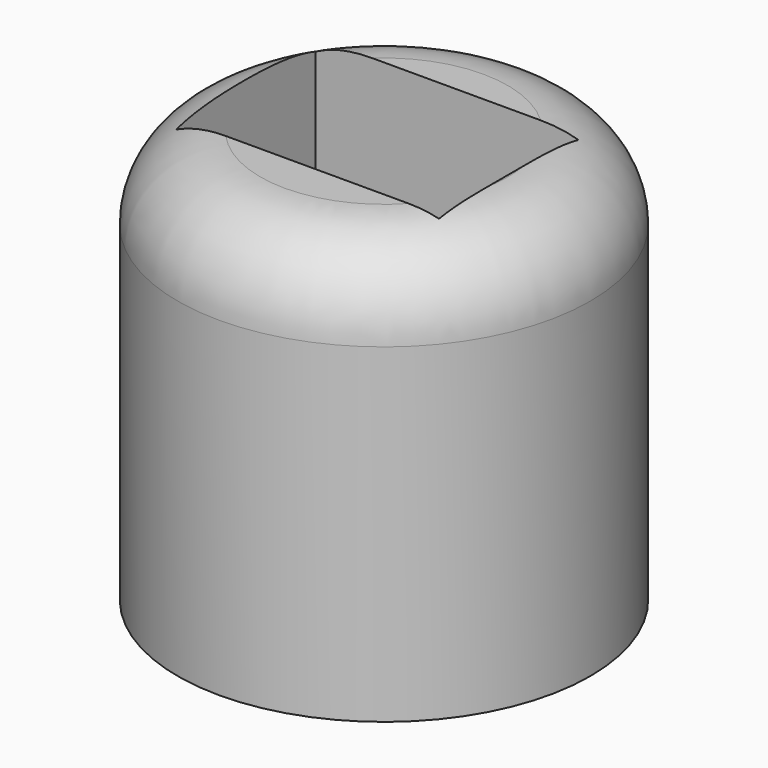
from build123d import *

# Parameters (mm, degrees)
F0_R     = 12.5
F1_DEPTH = 25
F2_W     = 15.9198134206
F2_H     = 10.5606685393
F3_DEPTH = 25


# Not quite as in the source:
# - a fillet or chamfer that OpenCascade refuses, or shapes differently, is made with other operations: its cross-section is extruded or revolved along the edge and cut away or added


with BuildPart() as f1:
    # F0 (on Top) → F1 (new body)
    with BuildSketch(Plane.XY):
        Circle(F0_R)
    extrude(amount=F1_DEPTH)

    # F2 (on face) → F3 (cut)
    with BuildSketch(Plane.XY.offset(25)):
        with Locations((-0.578898238, 0.2196121495)):
            Rectangle(F2_W, F2_H)
    extrude(amount=-F3_DEPTH, mode=Mode.SUBTRACT)

    # F4: fillet of radius 5 on 1 edges, made by hand

    # F4_s1 → F4_t2 (revolve, cut)
    with BuildSketch(Plane.XZ):
        with BuildLine():
            ThreePointArc((12.5, 20), (11.0355339059, 23.5355339059), (7.5, 25))
            Line((7.5, 25), (12.5, 25))
            Line((12.5, 25), (12.5, 20))
        make_face()
    revolve(axis=Axis((0, 0, 25), (0, 0, 1)), mode=Mode.SUBTRACT)


solid = f1.part
